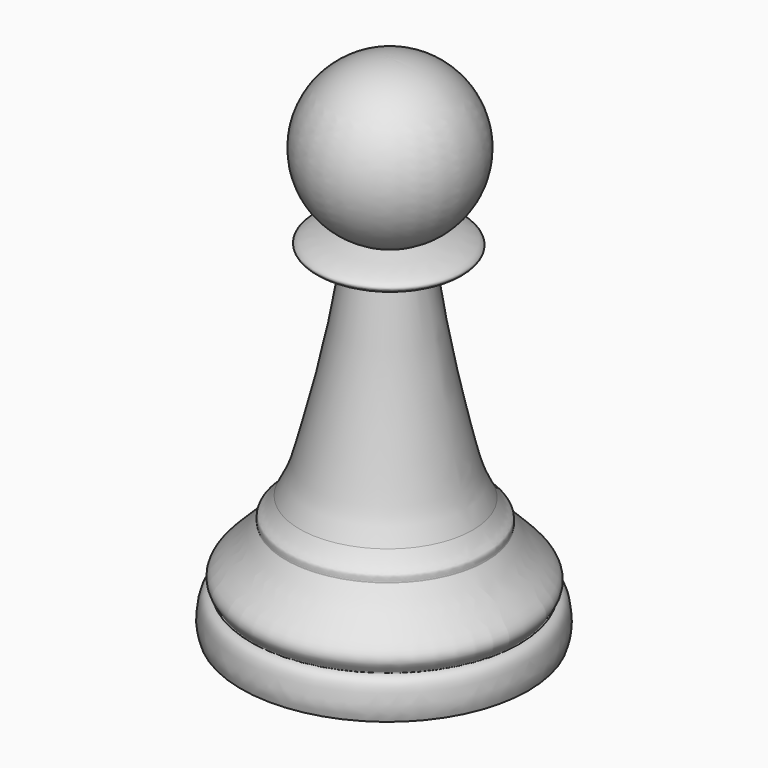
from build123d import *


with BuildPart() as f1:
    # F0 (on Front) → F1 (revolve)
    with BuildSketch(Plane.XZ):
        with BuildLine():
            add(Edge.make_bspline(
                [(-3.1662787523, 17.7566824135), (-2.5761022021, 17.6276873897), (-1.4496527783, 17.2948821281), (1.6836835905, 16.1425346039), (-1.5204735181, 14.8462763769), (-2.6737714204, 14.7152490292), (-3.2766132708, 14.6555562461)],
                knots=[0, 0, 0, 0, 0.2448530075, 0.4978909001, 0.75630568, 1, 1, 1, 1], degree=3))
            ThreePointArc((-3.1662787523, 17.7566824135), (1.0662747347, 26.9825385017), (-6.9088818999, 33.2616949922))
            Line((-6.9088818999, 33.2616949922), (-7.6604120992, -19.8863502592))
            Line((-7.6604120992, -19.8863502592), (7.3395879008, -19.8863502592))
            add(Edge.make_bspline(
                [(6.4222263949, -15.9084970219), (7.4382268502, -16.0586106128), (7.5445834117, -18.2973542943), (7.6678255333, -18.8182015492), (7.3395879008, -19.8863502592)],
                knots=[0.0101945625, 0.0101945625, 0.0101945625, 0.0101945625, 0.5201167763, 1, 1, 1, 1], degree=3))
            add(Edge.make_bspline(
                [(6.4222263949, -15.9084970219), (6.4087570306, -15.921420129), (5.9919830307, -16.0977828623), (7.4672570679, -14.7215623214), (5.774403452, -12.889064821), (4.4498110378, -11.6860957464), (3.335178552, -10.0726556153), (2.9579035472, -9.4817001373)],
                knots=[0.0085182385, 0.0085182385, 0.0085182385, 0.0085182385, 0.0188772342, 0.0996888693, 0.2116183545, 0.3387619974, 0.4043824956, 0.4043824956, 0.4043824956, 0.4043824956], degree=3))
            add(Edge.make_bspline(
                [(2.9579035472, -9.4817001373), (2.9504433345, -9.4732186482), (2.9443551758, -9.4634943718), (2.9394200334, -9.4527118784)],
                knots=[0, 0, 0, 0, 0.023159498, 0.023159498, 0.023159498, 0.023159498], degree=3))
            add(Edge.make_bspline(
                [(2.9394200334, -9.4527118784), (2.4539657662, -8.6904117345), (1.9730261393, -7.8605663495), (1.5695596727, -7.0848329195)],
                knots=[0.4054542345, 0.4054542345, 0.4054542345, 0.4054542345, 0.489908541, 0.489908541, 0.489908541, 0.489908541], degree=3))
            add(Edge.make_bspline(
                [(1.5695596727, -7.0848329195), (1.4151532471, -6.7879601034), (0.5716074491, -5.084192988), (-0.249737958, -1.8960238291), (-2.3399239854, 7.3761270189), (-3.2766132708, 14.6555562461)],
                knots=[0.489908541, 0.489908541, 0.489908541, 0.489908541, 0.522229164, 0.6804856824, 1, 1, 1, 1], degree=3))
        make_face()
        with BuildLine():
            add(Edge.make_bspline(
                [(2.9394200334, -9.4527118784), (2.906422235, -9.3806169895), (2.9478544009, -9.113916201), (2.8975432509, -8.7059428817), (2.2412513966, -8.3109123936), (1.6780537518, -7.2507213589), (1.5695596727, -7.0848329195)],
                knots=[0.023159498, 0.023159498, 0.023159498, 0.023159498, 0.1780106411, 0.3690348618, 0.6434842694, 1, 1, 1, 1], degree=3))
            add(Edge.make_bspline(
                [(2.9394200334, -9.4527118784), (2.4539657662, -8.6904117345), (1.9730261393, -7.8605663495), (1.5695596727, -7.0848329195)],
                knots=[0.4054542345, 0.4054542345, 0.4054542345, 0.4054542345, 0.489908541, 0.489908541, 0.489908541, 0.489908541], degree=3))
        make_face()
    revolve(axis=Axis((-7.2846469996, 0, 6.6876723665), (-0.0141389034, 0, -0.9999000407)))


solid = f1.part
